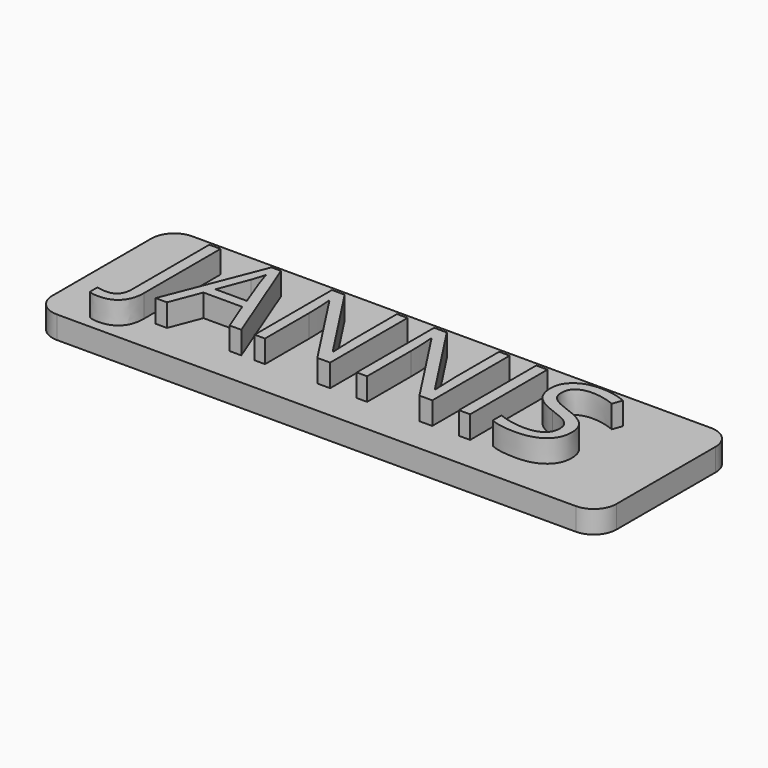
from build123d import *

# Parameters (mm, degrees)
F0_W         = 50
F0_H         = 15
F1_DEPTH     = 2
F2_TEXT_SIZE = 12.0108848644
F3_DEPTH     = 2
F4_R         = 2


# Not quite as in the source:
# - Text() gives the source's letters only with a copy of the font that has no kerning and outlines rounded to 1/6400 em; it was checked with that copy


with BuildPart() as f1:
    # F0 (on Top) → F1 (new body)
    with BuildSketch(Plane.XY):
        with Locations((4.5726578683, -6.3774778519)):
            Rectangle(F0_W, F0_H)
    extrude(amount=F1_DEPTH)

    # F2 (on face) → F3 (join)
    with BuildSketch(Plane.XY.offset(2)):
        with Locations((-15.4273421317, -10.7013964031)):
            Text('JANNIS', F2_TEXT_SIZE, font='Open Sans', text_align=(TextAlign.LEFT, TextAlign.BOTTOM))
    extrude(amount=F3_DEPTH)

    # F4
    f4_edges = [f1.edges().sort_by_distance(p)[0] for p in [
        (-20.427342, -13.877478, 1),
        (-20.427342, 1.122522, 1),
        (29.572658, -13.877478, 1),
        (29.572658, 1.122522, 1),
    ]]
    fillet(f4_edges, radius=F4_R)


solid = f1.part
